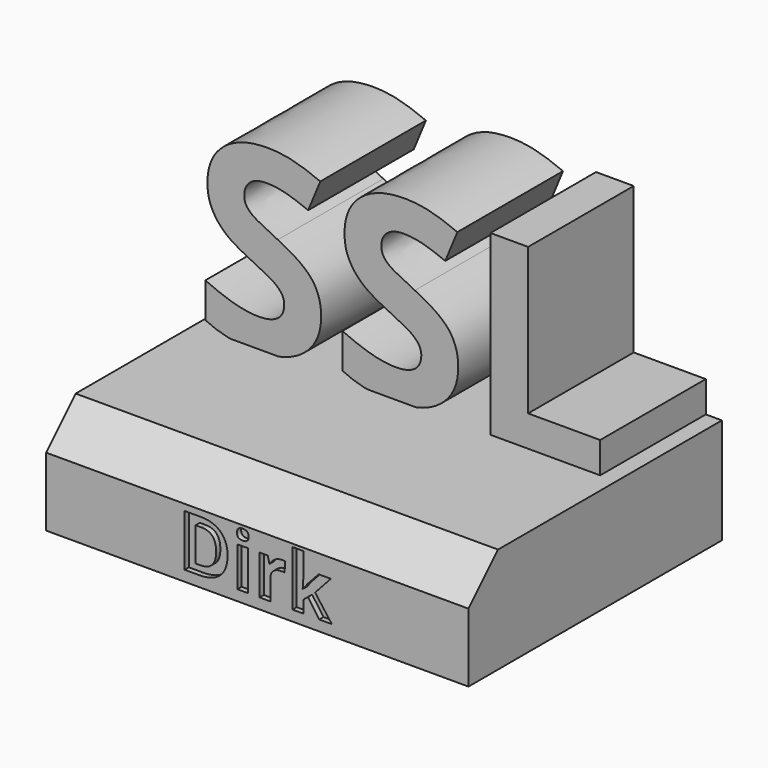
from build123d import *

# Parameters (mm, degrees)
F0_W         = 80
F0_H         = 60
F1_DEPTH     = 20
F2_TEXT_SIZE = 47.1368072178
F3_DEPTH     = 25
F4_SIZE      = 7
F5_TEXT_SIZE = 13.732923253
F6_DEPTH     = 1


# Not quite as in the source:
# - Text() gives the source's letters only with a copy of the font that has no kerning and outlines rounded to 1/6400 em; it was checked with that copy


with BuildPart() as f1:
    # F0 (on Top) → F1 (new body)
    with BuildSketch(Plane.XY):
        with Locations((0, -30)):
            Rectangle(F0_W, F0_H)
    extrude(amount=F1_DEPTH)

    # F4
    f4_edges = [f1.edges().sort_by_distance(p)[0] for p in [
        (0, -60, 20),
    ]]
    chamfer(f4_edges, length=F4_SIZE)

    # F5 (on face) → F6 (cut)
    with BuildSketch(Plane.XZ.offset(60)):
        with Locations((-15, 2)):
            Text('Dirk', F5_TEXT_SIZE, font='Open Sans', font_style=FontStyle.BOLD, text_align=(TextAlign.LEFT, TextAlign.BOTTOM))
    extrude(amount=-F6_DEPTH, mode=Mode.SUBTRACT)


with BuildPart() as f3:
    # F2 (on Front) → F3 (new body)
    with BuildSketch(Plane.XZ):
        with Locations((-40, 20)):
            Text('SSL', F2_TEXT_SIZE, font='Open Sans', font_style=FontStyle.BOLD, text_align=(TextAlign.LEFT, TextAlign.BOTTOM))
    extrude(amount=F3_DEPTH)


solid = Compound([f1.part, f3.part])
